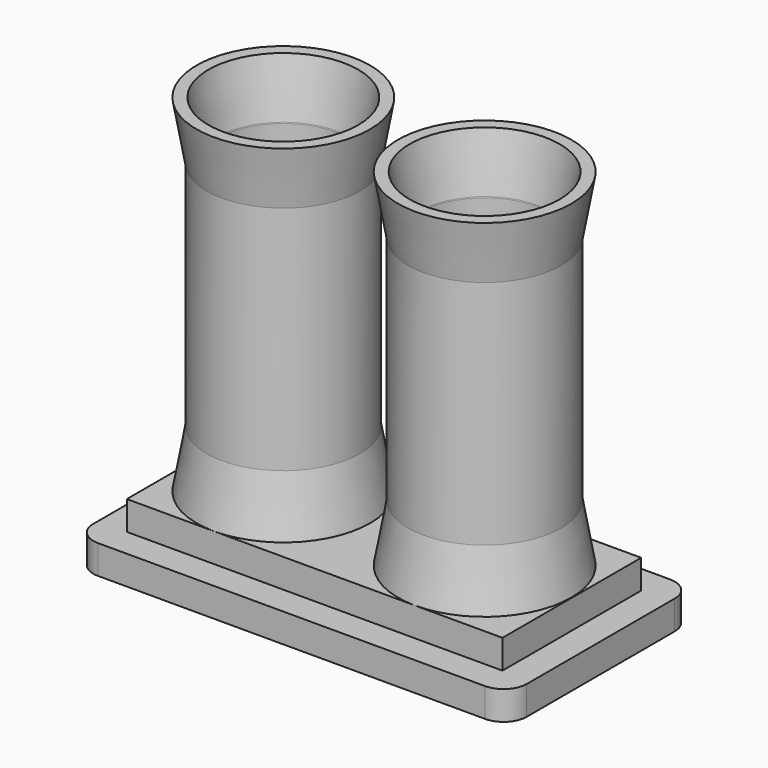
from build123d import *

# Parameters (mm, degrees)
F0_W         = 95.25
F0_H         = 50.8
F1_DEPTH     = 6.35
F2_W         = 82.55
F2_H         = 38.1
F3_DEPTH     = 6.35
F4_R         = 19.05
F5_DEPTH     = 12.7
F5_TAPER     = 10
F6_DEPTH     = 50.8
F6_FACE_R    = 16.810647345
F7_DEPTH     = 12.7
F7_TAPER     = -10
F8_T         = 2.54
F8_T3_DEPTH  = 87.63
F8_T5_DEPTH  = 43.18
F8_T8_ANGLE  = 180.0000001354
F8_T10_ANGLE = 90.000000001
F8_T12_ANGLE = 89.9999998666
F8_T14_ANGLE = 180.000000001
F8_T16_ANGLE = 90.000000001
F8_T18_ANGLE = 90.000000001
F9_R         = 5.08


# Not quite as in the source:
# - a shell that OpenCascade refuses in one call is made with other operations: the cavity is built on its own and cut out


with BuildPart() as f1:
    # F0 (on Top) → F1 (new body)
    with BuildSketch(Plane.XY):
        Rectangle(F0_W, F0_H)
    extrude(amount=F1_DEPTH)

    # F2 (on face) → F3 (join)
    with BuildSketch(Plane.XY.offset(6.35)):
        Rectangle(F2_W, F2_H)
    extrude(amount=F3_DEPTH)

    # F4 (on face) → F5 (join)
    with BuildSketch(Plane.XY.offset(12.7)):
        with Locations((-22.1206657588, 0)):
            Circle(F4_R)
        with Locations((22.1206657588, 0)):
            Circle(F4_R)
    extrude(amount=F5_DEPTH, taper=F5_TAPER)

    # F6 (add): faces of the model
    f6_faces = [f1.faces().sort_by_distance(p)[0] for p in [
        (-22.1206657588, 0, 25.4),
        (22.1206657588, 0, 25.4),
    ]]
    extrude(f6_faces, amount=F6_DEPTH)

    # F6_face (on face) → F7 (join)
    with BuildSketch(Plane(origin=(22.1206657588, 0, 76.2), x_dir=(1, 0, 0), z_dir=(0, 0, 1))):
        Circle(F6_FACE_R)
        with Locations((-44.2413315177, 0)):
            Circle(F6_FACE_R)
    extrude(amount=F7_DEPTH, taper=F7_TAPER)

    # F8: shell of thickness 2.54, made by hand


with BuildPart() as f8_core1:
    # F8_t2: copy of F1
    add(f1.part)

    # the walls: a layer under each face that stays
    f8_faces = [f8_core1.faces().sort_by_distance(p)[0] for p in [
        (0, -25.4, 3.175),
        (-47.625, 0, 3.175),
        (47.625, 0, 3.175),
        (-40.8214285714, -21.7714285714, 6.35),
        (0, 25.4, 3.175),
        (0, -19.05, 9.525),
        (41.275, 0, 9.525),
        (0, 19.05, 9.525),
        (-41.275, 0, 9.525),
        (-38.0826109524, -12.7, 12.7),
        (0, 0, 12.7),
        (38.0826109598, -12.7, 12.7),
        (-40.0509894313, 0, 19.05),
        (4.1903420863, 0, 19.05),
        (-38.9313131039, 0, 50.8),
        (5.3100184138, 0, 50.8),
        (-40.0509894313, 0, 82.55),
        (4.1903420863, 0, 82.55),
    ]]
    thicken(f8_faces, amount=-F8_T, mode=Mode.SUBTRACT)

    # F8_s4 → F8_t3 (cut)
    with BuildSketch(Plane.YZ.offset(-43.815)):
        Polygon((-19.0754, 6.3754), (-19.05, 3.81), (-16.51, 3.81), (-16.51, 6.35), align=None)
        Polygon((19.0754, 6.3754), (19.05, 3.81), (16.51, 3.81), (16.51, 6.35), align=None)
    extrude(amount=F8_T3_DEPTH, mode=Mode.SUBTRACT)

    # F8_s6 → F8_t5 (cut)
    with BuildSketch(Plane.XZ.offset(-21.59)):
        Polygon((41.3004, 6.3754), (41.275, 3.81), (38.735, 3.81), (38.735, 6.35), align=None)
        Polygon((-41.3004, 6.3754), (-41.275, 3.81), (-38.735, 3.81), (-38.735, 6.35), align=None)
    extrude(amount=F8_T5_DEPTH, mode=Mode.SUBTRACT)

    # F8_s7 → F8_t8 (revolve, cut)
    with BuildSketch(Plane.YZ.offset(-22.1206657588)):
        Polygon((-19.0750141169, 12.7298106637), (-19.05, 10.16), (-16.9186869368, 10.16), (-16.5485883073, 12.2589336287), align=None)
    revolve(axis=Axis((-22.1206657588, 0, 12.7), (0, 0, -1)), revolution_arc=F8_T8_ANGLE, mode=Mode.SUBTRACT)

    # F8_s9 → F8_t10 (revolve, cut)
    with BuildSketch(Plane.XZ):
        Polygon((-3.0456516419, 12.7298106637), (-3.0706657588, 10.16), (-5.201978822, 10.16), (-5.5720774515, 12.2589336287), align=None)
    revolve(axis=Axis((-22.1206657588, 0, 12.7), (0, 0, -1)), revolution_arc=F8_T10_ANGLE, mode=Mode.SUBTRACT)

    # F8_s11 → F8_t12 (revolve, cut)
    with BuildSketch(Plane.YZ.offset(-22.1206657588)):
        Polygon((19.0750141169, 12.7298106637), (19.05, 10.16), (16.9186869368, 10.16), (16.5485883073, 12.2589336287), align=None)
    revolve(axis=Axis((-22.1206657588, 0, 12.7), (0, 0, -1)), revolution_arc=F8_T12_ANGLE, mode=Mode.SUBTRACT)

    # F8_s13 → F8_t14 (revolve, cut)
    with BuildSketch(Plane.YZ.offset(22.1206657588)):
        Polygon((-19.0750141169, 12.7298106637), (-19.05, 10.16), (-16.9186869368, 10.16), (-16.5485883073, 12.2589336287), align=None)
    revolve(axis=Axis((22.1206657588, 0, 12.7), (0, 0, -1)), revolution_arc=F8_T14_ANGLE, mode=Mode.SUBTRACT)

    # F8_s15 → F8_t16 (revolve, cut)
    with BuildSketch(Plane.XZ):
        Polygon((41.1956798758, 12.7298106637), (41.1706657588, 10.16), (39.0393526957, 10.16), (38.6692540662, 12.2589336287), align=None)
    revolve(axis=Axis((22.1206657588, 0, 12.7), (0, 0, -1)), revolution_arc=F8_T16_ANGLE, mode=Mode.SUBTRACT)

    # F8_s17 → F8_t18 (revolve, cut)
    with BuildSketch(Plane.YZ.offset(22.1206657588)):
        Polygon((19.0750141169, 12.7298106637), (19.05, 10.16), (16.9186869368, 10.16), (16.5485883073, 12.2589336287), align=None)
    revolve(axis=Axis((22.1206657588, 0, 12.7), (0, 0, -1)), revolution_arc=F8_T18_ANGLE, mode=Mode.SUBTRACT)

    # F8_s19 → F8_t20 (revolve, cut)
    with BuildSketch(Plane.XZ):
        Polygon((-5.2596042969, 25.4044106637), (-7.8114301065, 24.9589336287), (-7.8500184138, 25.1777787946), (-7.8500184138, 25.4), align=None)
    revolve(axis=Axis((-22.1206657588, 0, 25.4), (0, 0, -1)), mode=Mode.SUBTRACT)

    # F8_s21 → F8_t22 (revolve, cut)
    with BuildSketch(Plane.XZ):
        Polygon((38.9817272208, 25.4044106637), (36.4299014112, 24.9589336287), (36.3913131039, 25.1777787946), (36.3913131039, 25.4), align=None)
    revolve(axis=Axis((22.1206657588, 0, 25.4), (0, 0, -1)), mode=Mode.SUBTRACT)

    # F8_s23 → F8_t24 (revolve, cut)
    with BuildSketch(Plane.XZ):
        Polygon((-5.2596042969, 76.1955893363), (-7.8500184138, 76.2), (-7.8500184138, 76.4222212054), (-7.8114301065, 76.6410663713), align=None)
    revolve(axis=Axis((-22.1206657588, 0, 76.2), (0, 0, -1)), mode=Mode.SUBTRACT)

    # F8_s25 → F8_t26 (revolve, cut)
    with BuildSketch(Plane.XZ):
        Polygon((38.9817272208, 76.1955893363), (36.3913131039, 76.2), (36.3913131039, 76.4222212054), (36.4299014112, 76.6410663713), align=None)
    revolve(axis=Axis((22.1206657588, 0, 76.2), (0, 0, -1)), mode=Mode.SUBTRACT)


with BuildPart() as f1_1:
    add(f1.part)

    # what is left inside the walls is the cavity
    f8_cavity = [f8_core1.part.solids().sort_by_distance(p)[0] for p in [
        (-36.365913, 0, 59.266667),
    ]]
    add(f8_cavity, mode=Mode.SUBTRACT)

    # F9
    f9_edges = [f1_1.edges().sort_by_distance(p)[0] for p in [
        (-47.625, -25.4, 3.175),
        (47.625, -25.4, 3.175),
        (47.625, 25.4, 3.175),
        (-47.625, 25.4, 3.175),
    ]]
    fillet(f9_edges, radius=F9_R)


solid = f1_1.part
